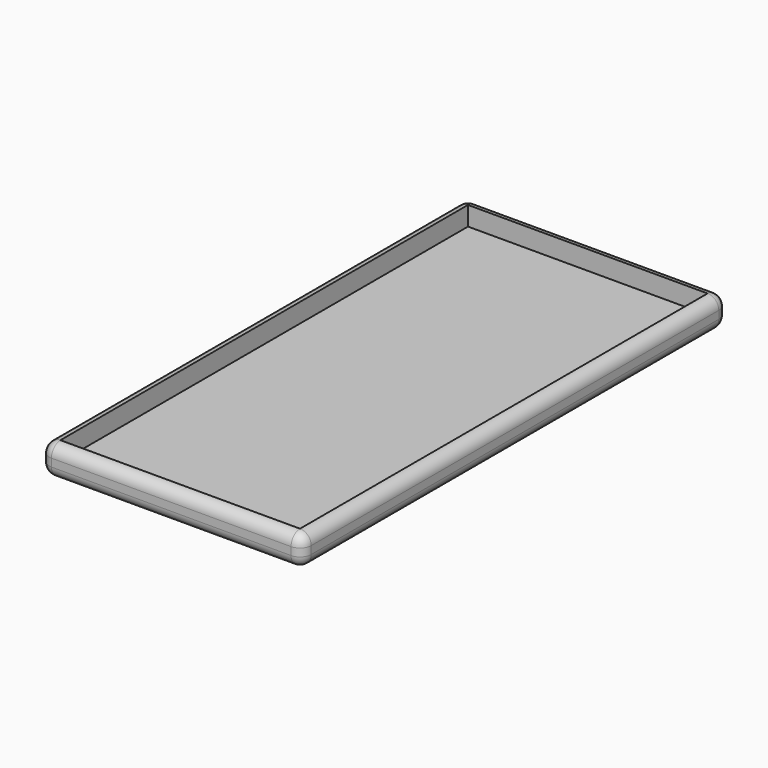
from build123d import *

# Parameters (mm, degrees)
F0_W     = 70.1
F0_H     = 142.3
F1_DEPTH = 8.1
F2_T     = -3
F3_R     = 2.99999


# Not quite as in the source:
# - a fillet or chamfer is up to 0.001 mm smaller than in the source, because OpenCascade refuses the exact size


with BuildPart() as f1:
    # F0 (on Top) → F1 (new body)
    with BuildSketch(Plane.XY):
        Rectangle(F0_W, F0_H)
    extrude(amount=F1_DEPTH)

    # F2
    f2_openings = [f1.faces().sort_by_distance(p)[0] for p in [
        (0, 0, 8.1),
    ]]
    offset(amount=F2_T, openings=f2_openings)

    # F3 (radius 3 in the source; OpenCascade refuses exactly that, so slightly less here)
    f3_edges = [f1.edges().sort_by_distance(p)[0] for p in [
        (-35.05, -71.15, 4.05),
        (35.05, -71.15, 4.05),
        (0, -71.15, 0),
        (0, -71.15, 8.1),
        (35.05, 71.15, 4.05),
        (35.05, 0, 0),
        (35.05, 0, 8.1),
        (-35.05, 71.15, 4.05),
        (0, 71.15, 0),
        (0, 71.15, 8.1),
        (-35.05, 0, 0),
        (-35.05, 0, 8.1),
    ]]
    fillet(f3_edges, radius=F3_R)


solid = f1.part
